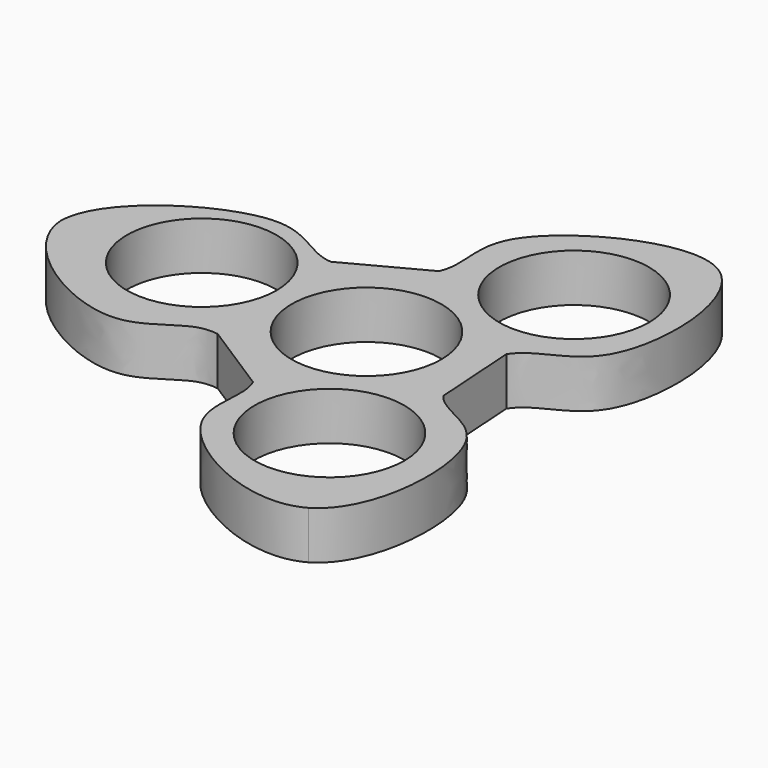
from build123d import *

# Parameters (mm, degrees)
F0_R     = 10.925
F1_DEPTH = 7


with BuildPart() as f1:
    # F0 (on Top) → F1 (new body)
    with BuildSketch(Plane.XY):
        with BuildLine():
            add(Edge.make_bspline(
                [(-6.4395543964, 13.2348172529), (-9.1292198143, 12.2456790048), (-11.7414815686, 11.1713296384), (-13.9497888892, 11.3483672356)],
                knots=[0.1400697691, 0.1400697691, 0.1400697691, 0.1400697691, 0.3121200653, 0.3121200653, 0.3121200653, 0.3121200653], degree=3))
            add(Edge.make_bspline(
                [(-13.9497888892, 11.3483672356), (-17.5573593522, 11.6375822379), (-23.7480393822, 20.5188284103), (-44.3087168864, 7.5057952096), (-44.2924838881, 0)],
                knots=[0.3121200653, 0.3121200653, 0.3121200653, 0.3121200653, 0.5931876328, 1, 1, 1, 1], degree=3))
            add(Edge.make_bspline(
                [(-12.887299612, -10.6033772899), (-13.4512132627, -10.5222545013), (-17.6938513535, -10.3298112003), (-23.4895130797, -20.2738643689), (-43.8788694911, -7.371346434), (-44.2924838881, 0)],
                knots=[0.278216512, 0.278216512, 0.278216512, 0.278216512, 0.3185350392, 0.5938778395, 0.9927419326, 0.9927419326, 0.9927419326, 0.9927419326], degree=3))
            add(Edge.make_bspline(
                [(-7.0311428775, -12.4986186093), (-9.0891121607, -11.6866108154), (-11.0989087543, -10.8606493977), (-12.887299612, -10.6033772899)],
                knots=[0.1503506848, 0.1503506848, 0.1503506848, 0.1503506848, 0.278216512, 0.278216512, 0.278216512, 0.278216512], degree=3))
            add(Edge.make_bspline(
                [(-7.0311428775, -12.4986186093), (-5.0355845098, -14.0840137015), (-3.1635826547, -15.6293105857), (-2.3408499564, -17.3583158347)],
                knots=[0.1677034297, 0.1677034297, 0.1677034297, 0.1677034297, 0.3163832996, 0.3163832996, 0.3163832996, 0.3163832996], degree=3))
            add(Edge.make_bspline(
                [(-2.3408499564, -17.3583158347), (-2.327038362, -17.3873414455), (-0.8208991693, -20.6275709181), (-6.2778244318, -30.204015976), (15.5191329345, -41.4031973523), (21.9899696205, -37.6485751695)],
                knots=[0.3163832996, 0.3163832996, 0.3163832996, 0.3163832996, 0.3188792574, 0.594519601, 1, 1, 1, 1], degree=3))
            add(Edge.make_bspline(
                [(16.7283741857, -6.4672911408), (18.786584329, -9.3376357175), (29.6744078467, -9.4662536369), (28.481763025, -33.9192331377), (21.9899696205, -37.6485751695)],
                knots=[0.3188786975, 0.3188786975, 0.3188786975, 0.3188786975, 0.5942210158, 1, 1, 1, 1], degree=3))
            add(Edge.make_bspline(
                [(14.5053291097, 1.8450627629), (15.0185483744, -1.3196723959), (15.3415537221, -4.5332551), (16.7283741857, -6.4672911408)],
                knots=[0.1333532483, 0.1333532483, 0.1333532483, 0.1333532483, 0.3188786975, 0.3188786975, 0.3188786975, 0.3188786975], degree=3))
            add(Edge.make_bspline(
                [(14.5053291097, 1.8450627629), (14.8069082277, 3.4605447135), (15.20732089, 4.9267216062), (15.9087433766, 6.0301086055)],
                knots=[0.2104833034, 0.2104833034, 0.2104833034, 0.2104833034, 0.3108563735, 0.3108563735, 0.3108563735, 0.3108563735], degree=3))
            add(Edge.make_bspline(
                [(15.9087433766, 6.0301086055), (15.9624030761, 6.1145190941), (18.0051316038, 9.1474766545), (29.1059131262, 9.1929649799), (27.9873138953, 33.8233167393), (21.4900302358, 37.5558127591)],
                knots=[0.3108563735, 0.3108563735, 0.3108563735, 0.3108563735, 0.3185350392, 0.5938778395, 1, 1, 1, 1], degree=3))
            add(Edge.make_bspline(
                [(-2.8908584222, 17.2268748699), (-1.431266538, 20.4410048292), (-6.8808579099, 29.9699369249), (15.0089520333, 41.316377454), (21.4900302358, 37.5558127591)],
                knots=[0.3185350392, 0.3185350392, 0.3185350392, 0.3185350392, 0.5938778395, 1, 1, 1, 1], degree=3))
            add(Edge.make_bspline(
                [(-6.4395543964, 13.2348172529), (-4.8831854727, 14.5225004957), (-3.5328470445, 15.8131681433), (-2.8908584222, 17.2268748699)],
                knots=[0.197427936, 0.197427936, 0.197427936, 0.197427936, 0.3185350392, 0.3185350392, 0.3185350392, 0.3185350392], degree=3))
        make_face()
        with Locations((12.3414872441, -21.7546906004)):
            Circle(F0_R, mode=Mode.SUBTRACT)
        with Locations((0.018236467, 0.3984128004)):
            Circle(F0_R, mode=Mode.SUBTRACT)
        with Locations((-25.2826381154, 1.9758301096)):
            Circle(F0_R, mode=Mode.SUBTRACT)
        with Locations((12.7906060968, 22.2956517596)):
            Circle(F0_R, mode=Mode.SUBTRACT)
        with BuildLine():
            Line((-2.8908584222, 17.2268748699), (-13.9497888892, 11.3483672356))
            add(Edge.make_bspline(
                [(-6.4395543964, 13.2348172529), (-9.1292198143, 12.2456790048), (-11.7414815686, 11.1713296384), (-13.9497888892, 11.3483672356)],
                knots=[0.1400697691, 0.1400697691, 0.1400697691, 0.1400697691, 0.3121200653, 0.3121200653, 0.3121200653, 0.3121200653], degree=3))
            add(Edge.make_bspline(
                [(-6.4395543964, 13.2348172529), (-4.8831854727, 14.5225004957), (-3.5328470445, 15.8131681433), (-2.8908584222, 17.2268748699)],
                knots=[0.197427936, 0.197427936, 0.197427936, 0.197427936, 0.3185350392, 0.3185350392, 0.3185350392, 0.3185350392], degree=3))
        make_face()
        with BuildLine():
            add(Edge.make_bspline(
                [(-7.0311428775, -12.4986186093), (-9.0891121607, -11.6866108154), (-11.0989087543, -10.8606493977), (-12.887299612, -10.6033772899)],
                knots=[0.1503506848, 0.1503506848, 0.1503506848, 0.1503506848, 0.278216512, 0.278216512, 0.278216512, 0.278216512], degree=3))
            Line((-12.887299612, -10.6033772899), (-2.3408499564, -17.3583158347))
            add(Edge.make_bspline(
                [(-7.0311428775, -12.4986186093), (-5.0355845098, -14.0840137015), (-3.1635826547, -15.6293105857), (-2.3408499564, -17.3583158347)],
                knots=[0.1677034297, 0.1677034297, 0.1677034297, 0.1677034297, 0.3163832996, 0.3163832996, 0.3163832996, 0.3163832996], degree=3))
        make_face()
        with BuildLine():
            Line((16.7283741857, -6.4672911408), (15.9087433766, 6.0301086055))
            add(Edge.make_bspline(
                [(14.5053291097, 1.8450627629), (14.8069082277, 3.4605447135), (15.20732089, 4.9267216062), (15.9087433766, 6.0301086055)],
                knots=[0.2104833034, 0.2104833034, 0.2104833034, 0.2104833034, 0.3108563735, 0.3108563735, 0.3108563735, 0.3108563735], degree=3))
            add(Edge.make_bspline(
                [(14.5053291097, 1.8450627629), (15.0185483744, -1.3196723959), (15.3415537221, -4.5332551), (16.7283741857, -6.4672911408)],
                knots=[0.1333532483, 0.1333532483, 0.1333532483, 0.1333532483, 0.3188786975, 0.3188786975, 0.3188786975, 0.3188786975], degree=3))
        make_face()
    extrude(amount=F1_DEPTH)


solid = f1.part
